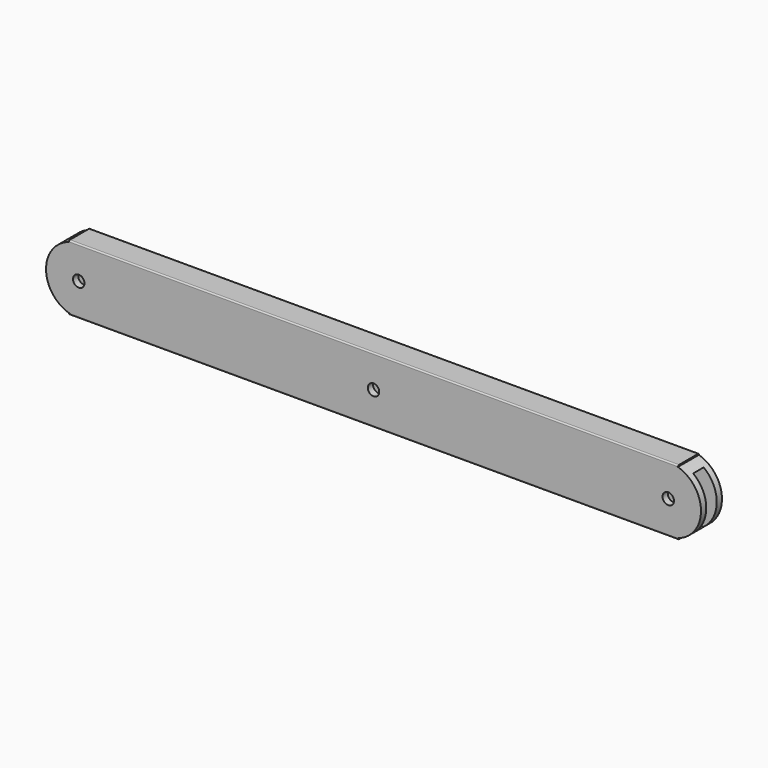
from build123d import *

# Parameters (mm, degrees)
F3_W     = 20
F3_H     = 80
F4_DEPTH = 500
F6_D     = 17.5
F6_DEPTH = 40
F6_TIP   = 5.2575304165
F7_DEPTH = 40
F8_DEPTH = 35
F9_DEPTH = 35


# Not quite as in the source:
# - a feature names something its author has since deleted; it is built from what else it names


with BuildPart() as f4:
    # F3 (on Right) → F4 (new body, symmetric)
    with BuildSketch(Plane.YZ):
        with BuildLine():
            ThreePointArc((-4.2945303673, -84.5), (-3.7087439297, -85.9142135624), (-2.2945303673, -86.5))
            Line((-2.2945303673, -86.5), (33.7054696327, -86.5))
            ThreePointArc((33.7054696327, -86.5), (35.1196831951, -85.9142135624), (35.7054696327, -84.5))
            Line((35.7054696327, -84.5), (35.7054696327, 11.5))
            ThreePointArc((35.7054696327, 11.5), (35.1196831951, 12.9142135624), (33.7054696327, 13.5))
            Line((33.7054696327, 13.5), (-2.2945303673, 13.5))
            ThreePointArc((-2.2945303673, 13.5), (-3.7087439297, 12.9142135624), (-4.2945303673, 11.5))
            Line((-4.2945303673, 11.5), (-4.2945303673, -84.5))
        make_face()
        with Locations((15.7054696327, -36.5)):
            Rectangle(F3_W, F3_H, mode=Mode.SUBTRACT)
    extrude(amount=F4_DEPTH, both=True)

    # F6
    with Locations(Plane.XZ.offset(4.2945303673)):
        with Locations((450, -36.2195856869), (0, -36.2195856869), (-450, -36.5)):
            Hole(F6_D / 2, depth=F6_DEPTH)
            with Locations((0, 0, -(F6_DEPTH + F6_TIP / 2))):  # 118° drill point
                Cone(0, F6_D / 2, F6_TIP, mode=Mode.SUBTRACT)

    # F5 (on face) → F7 (cut)
    with BuildSketch(Plane.XZ.offset(4.2945303673)):
        with BuildLine():
            ThreePointArc((-500, -36.5), (-490, -6.5), (-464, 11.5))
            Line((-464, 11.5), (-500, 11.5))
            Line((-500, 11.5), (-500, -36.5))
        make_face()
        with BuildLine():
            ThreePointArc((-464, -84.5), (-490, -66.5), (-500, -36.5))
            Line((-500, -36.5), (-500, -84.5))
            Line((-500, -84.5), (-464, -84.5))
        make_face()
        with BuildLine():
            Line((500, 11.5), (464, 11.5))
            ThreePointArc((464, 11.5), (490, -6.5), (500, -36.5))
            Line((500, -36.5), (500, 11.5))
        make_face()
        with BuildLine():
            Line((500, -84.5), (500, -36.5))
            ThreePointArc((500, -36.5), (490, -66.5), (464, -84.5))
            Line((464, -84.5), (500, -84.5))
        make_face()
    extrude(amount=-F7_DEPTH, mode=Mode.SUBTRACT)

    # F8 (cut): faces of the model
    f8_faces = [f4.faces().sort_by_distance(p)[0] for p in [
        (-500, 15.7054696327, 12.4878664624),
        (-500, 15.7054696327, -85.4878664624),
    ]]
    extrude(f8_faces, amount=-F8_DEPTH, mode=Mode.SUBTRACT)

    # F9 (cut): faces of the model
    f9_faces = [f4.faces().sort_by_distance(p)[0] for p in [
        (500, 15.7054696327, -85.4878664624),
        (500, 15.7054696327, 12.4878664624),
    ]]
    extrude(f9_faces, amount=-F9_DEPTH, mode=Mode.SUBTRACT)


solid = f4.part
